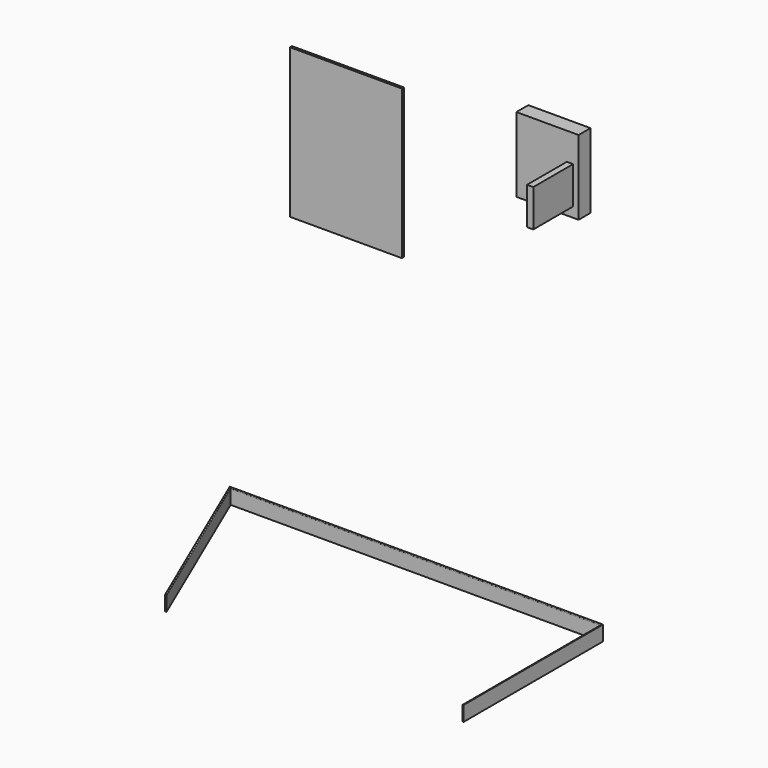
from build123d import *

# Parameters (mm, degrees)
F3_W      = 5
F3_H      = 60
F5_R      = 3
F6_W      = 250
F6_H      = 300
F7_DEPTH  = 60
F8_W      = 200
F8_H      = 150
F9_DEPTH  = 25
F10_W     = 450
F10_H     = 600
F11_DEPTH = 10


with BuildPart() as f4:
    # F4: sweep along a path in F0
    with BuildLine(Plane.XY) as f4_path:
        Line((1426.8305338016, -639.3725686498), (1426.8305338016, 55.6274313502))
        Line((1426.8305338016, 55.6274313502), (-60.5867711228, 55.6274313502))
        Line((-60.5867711228, 55.6274313502), (236.4262589517, -637.4029721569))
    # F3 (on line) → F4 (sweep)
    with BuildSketch(Plane.XZ.offset(639.3725686498)):
        with Locations((1429.3305338016, 30)):
            Rectangle(F3_W, F3_H)
    sweep(path=f4_path.line, transition=Transition.RIGHT)

    # F5
    f5_edges = [f4.edges().sort_by_distance(p)[0] for p in [
        (1426.830534, -291.872569, 60),
        (683.121881, 55.627431, 60),
        (87.919744, -290.88777, 60),
    ]]
    fillet(f5_edges, radius=F5_R)


with BuildPart() as f7:
    # F6 (on face) → F7 (new body)
    with BuildSketch(Plane.XZ.offset(-60.6274313502)):
        with Locations((1256.8305338016, 1650)):
            Rectangle(F6_W, F6_H)
    extrude(amount=F7_DEPTH)


with BuildPart() as f9:
    # F8 (on face) → F9 (new body)
    with BuildSketch(Plane(origin=(1431.8305338016, 0, 0), x_dir=(0, -1, 0), z_dir=(-1, 0, 0))):
        with Locations((189.3725686498, 1675)):
            Rectangle(F8_W, F8_H)
    extrude(amount=F9_DEPTH)


with BuildPart() as f11:
    # F10 (on face) → F11 (new body)
    with BuildSketch(Plane.XZ.offset(-60.6274313502)):
        with Locations((406.8305338016, 1400)):
            Rectangle(F10_W, F10_H)
    extrude(amount=F11_DEPTH)


solid = Compound([f4.part, f7.part, f9.part, f11.part])
